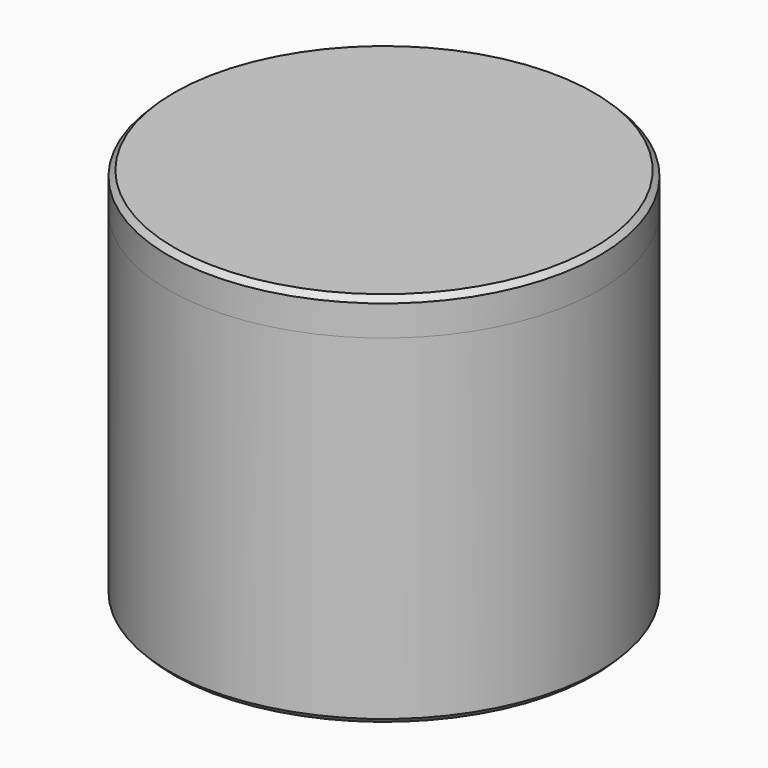
from build123d import *

# Parameters (mm, degrees)
F0_W    = 20
F0_H    = 10
F0_W_2  = 5
F4_SIZE = 1.5
F5_SIZE = 1.5


# Not quite as in the source:
# - a feature names something its author has since deleted; it is built from what else it names


with BuildPart() as f1:
    # F0 (on Front) → F1 (revolve)
    with BuildSketch(Plane.XZ):
        Polygon((-60, 45), (-60, 35), (-45, 35), (-45, 45), (-50, 45), align=None)
        Polygon((-60, -45), (0, -45), (0, -35), (-25, -35), (-25, 15), (-45, 35), (-60, 35), align=None)
        Polygon((-55, 50), (-60, 50), (-60, 45), (-50, 45), align=None)
    revolve(axis=Axis((0, 0, 13.6922076344), (0, 0, -1)))

    # F5
    f5_edges = [f1.edges().sort_by_distance(p)[0] for p in [
        (60, 0, -45),
    ]]
    chamfer(f5_edges, length=F5_SIZE)


with BuildPart() as f2:
    # F0 (on Front) → F2 (revolve)
    with BuildSketch(Plane.XZ):
        Polygon((0, -30), (0, 35), (-20, 35), (-20, 30), (-20, -30), align=None)
        with Locations((-10, 40)):
            Rectangle(F0_W, F0_H)
        Polygon((0, 45), (0, 60), (-60, 60), (-60, 50), (-55, 50), (-50, 45), (-45, 45), (-25, 45), (-20, 45), align=None)
    revolve(axis=Axis((0, 0, 13.6922076344), (0, 0, -1)))

    # F4
    f4_edges = [f2.edges().sort_by_distance(p)[0] for p in [
        (60, 0, 60),
    ]]
    chamfer(f4_edges, length=F4_SIZE)


with BuildPart() as f3:
    # F0 (on Front) → F3 (revolve)
    with BuildSketch(Plane.XZ):
        with Locations((-35, 40)):
            Rectangle(F0_W, F0_H)
        with Locations((-22.5, 40)):
            Rectangle(F0_W_2, F0_H)
        Polygon((-25, -35), (0, -35), (0, -30), (-20, -30), (-20, 30), (-20, 35), (-25, 35), (-25, 15), align=None)
        Polygon((-25, 35), (-45, 35), (-25, 15), align=None)
    revolve(axis=Axis((0, 0, 13.6922076344), (0, 0, -1)))


solid = Compound([f1.part, f2.part, f3.part])
